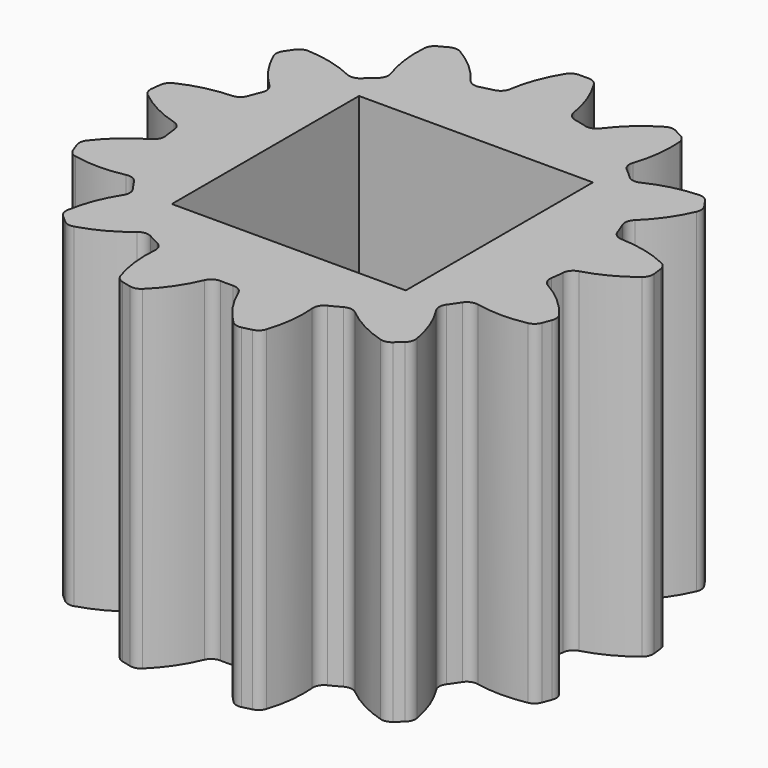
from build123d import *

# Parameters (mm, degrees)
F0_W            = 4.2
F0_H            = 4.2
F1_DEPTH        = 6
F2_DEPTH        = 6
F2_COPIES_COUNT = 13
F3_R            = 0.2


# Not quite as in the source:
# - a pattern or mirror of a feature is missing from the dataset's text; its kind, count and spacing are read off the source's solid
# - a feature names something its author has since deleted; it is built from what else it names


with BuildPart() as f1:
    # F0 (on Top) → F1 (new body)
    with BuildSketch(Plane.XY):
        with BuildLine():
            ThreePointArc((-0.5925235657, 3.4494805151), (-2.2556781153, -2.6761756744), (3.5, 0))
            ThreePointArc((3.5, 0), (2.6729076381, 2.2595496804), (0.582534424, 3.4511814854))
            ThreePointArc((0.582534424, 3.4511814854), (-0.0050664645, 3.499996333), (-0.5925235657, 3.4494805151))
        make_face()
        Rectangle(F0_W, F0_H, mode=Mode.SUBTRACT)
    extrude(amount=F1_DEPTH)

    # F0 (on Top) → F2 (join)
    with BuildSketch(Plane.XY):
        with BuildLine():
            ThreePointArc((-0.5925235657, 3.4494805151), (-0.0050664645, 3.499996333), (0.582534424, 3.4511814854))
            ThreePointArc((0.582534424, 3.4511814854), (0.4545899807, 4.0153836344), (0.1870099374, 4.5283112764))
            Line((0.1870099374, 4.5283112764), (-0.1973801256, 4.5283112764))
            ThreePointArc((-0.1973801256, 4.5283112764), (-0.4650844032, 4.0145833539), (-0.5925235657, 3.4494805151))
        make_face()
    f2 = extrude(amount=F2_DEPTH)

    # F2_copies: F2 ×13 about axis
    f2_copies_axis = Axis((0, 0, 0), (0, 0, 1))
    for i in range(1, F2_COPIES_COUNT):
        add(f2.rotate(f2_copies_axis, i * 360 / F2_COPIES_COUNT))

    # F3
    f3_edges = [f1.edges().sort_by_distance(p)[0] for p in [
        (-0.19738, 4.528311, 3),
        (0.18701, 4.528311, 3),
        (3.435432, -0.669183, 3),
        (3.496235, -0.162293, 3),
        (4.304037, -1.421208, 3),
        (4.517836, 0.360181, 3),
        (4.471503, 0.741769, 3),
        (3.352909, 1.003992, 3),
        (3.171184, 1.481078, 3),
        (3.832961, 2.418468, 3),
        (3.614602, 2.734815, 3),
        (2.502275, 2.447166, 3),
        (0.582534, 3.451181, 3),
        (1.0784, 3.329723, 3),
        (2.119653, 2.785152, 3),
        (-0.592524, 3.449481, 3),
        (-1.088035, 3.326587, 3),
        (-1.938822, 4.096528, 3),
        (-2.279183, 3.917893, 3),
        (-2.127707, 2.779004, 3),
        (-2.509349, 2.439911, 3),
        (-3.620493, 2.72628, 3),
        (-3.838852, 2.409933, 3),
        (-3.175459, 1.471891, 3),
        (-3.355802, 0.994281, 3),
        (-4.472753, 0.731474, 3),
        (-4.519086, 0.349887, 3),
        (-3.495751, -0.172414, 3),
        (-3.43348, -0.679127, 3),
        (-4.300359, -1.430904, 3),
        (-4.164053, -1.790315, 3),
        (-3.015209, -1.777222, 3),
        (-2.72459, -2.196955, 3),
        (-3.142805, -3.265479, 3),
        (-2.855085, -3.520377, 3),
        (-1.843918, -2.974889, 3),
        (-1.391529, -3.211487, 3),
        (-1.265272, -4.351972, 3),
        (-0.892051, -4.443963, 3),
        (-0.250209, -3.491045, 3),
        (0.260315, -3.490306, 3),
        (0.90212, -4.441481, 3),
        (1.27534, -4.349491, 3),
        (1.400821, -3.207445, 3),
        (1.852523, -2.969538, 3),
        (2.862847, -3.5135, 3),
        (3.150567, -3.258602, 3),
        (2.730939, -2.189057, 3),
        (3.020341, -1.768485, 3),
        (4.16773, -1.780619, 3),
        (1.92964, 4.101348, 3),
        (2.27, 3.922713, 3),
    ]]
    fillet(f3_edges, radius=F3_R)


solid = f1.part
